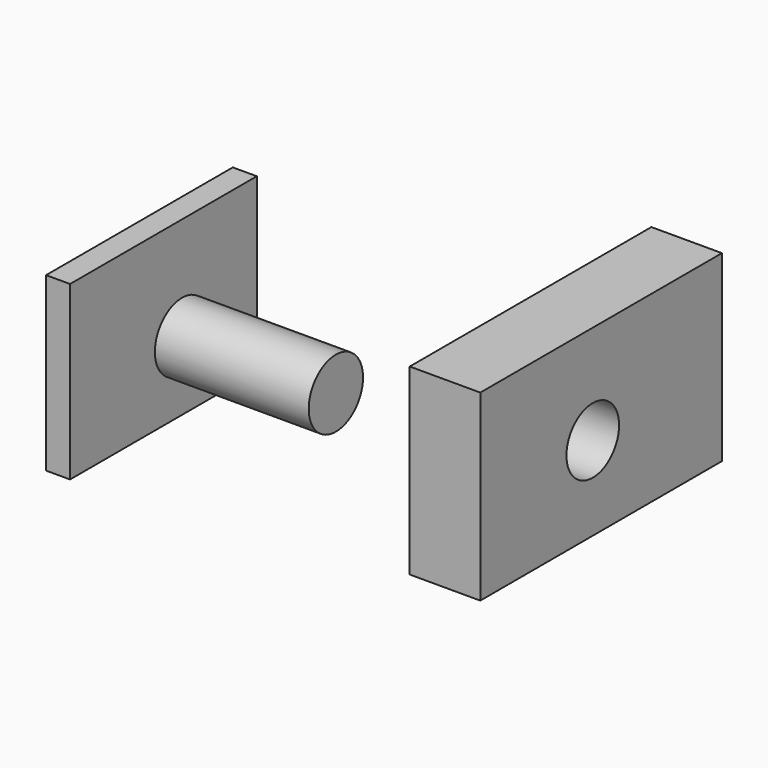
from build123d import *

# Parameters (mm, degrees)
F3_W     = 84.005985409
F3_H     = 61.9537178427
F3_R     = 9.2521212974
F4_DEPTH = 8.636
F5_R     = 12.2230702702
F6_DEPTH = 55.372
F7_W     = 108.715981245
F7_H     = 65.9279860556
F7_R     = 11.8387821777
F8_DEPTH = 25.4


# Not quite as in the source:
# - the program builds the solid bodies; features that only make, move or delete a surface that nothing else refers to are left out


with BuildPart() as f4:
    # F3 (on face) → F4 (new body)
    with BuildSketch(Plane.YZ):
        with Locations((-8.3795879036, 9.0704439208)):
            Rectangle(F3_W, F3_H)
        with Locations((0, 2.9850138817)):
            Circle(F3_R, mode=Mode.SUBTRACT)
    extrude(amount=F4_DEPTH)

    # F5 (on face) → F6 (join)
    with BuildSketch(Plane.YZ.offset(8.636)):
        with Locations((0, 2.9850138817)):
            Circle(F5_R)
    extrude(amount=F6_DEPTH)


with BuildPart() as f8:
    # F7 (on Right) → F8 (new body)
    with BuildSketch(Plane.YZ):
        with Locations((167.6053851843, -88.389961049)):
            Rectangle(F7_W, F7_H)
        with Locations((163.8479083776, -91.1392197013)):
            Circle(F7_R, mode=Mode.SUBTRACT)
    extrude(amount=F8_DEPTH)


solid = Compound([f4.part, f8.part])
